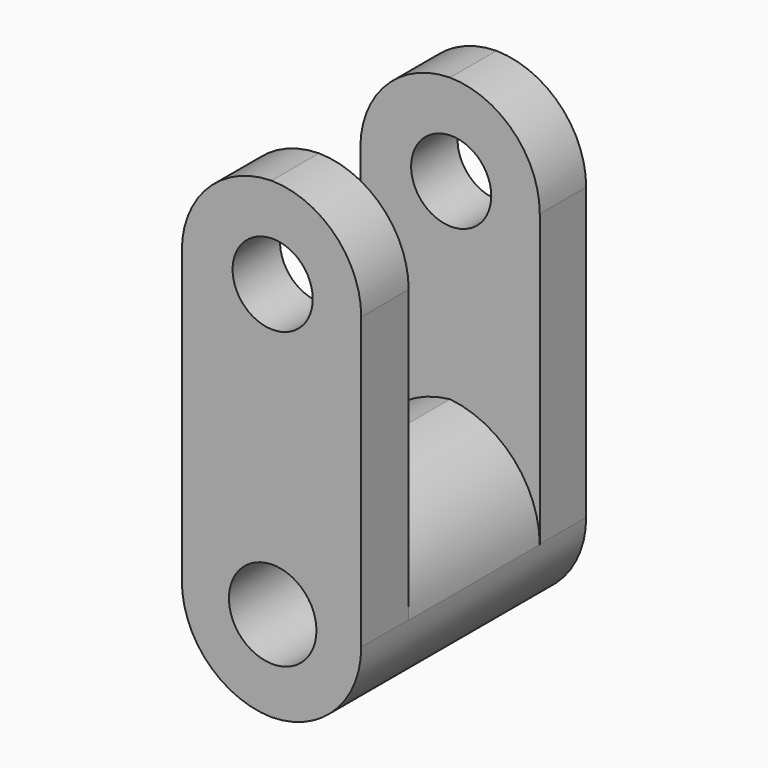
from build123d import *

# Parameters (mm, degrees)
F0_W        = 58.9435696602
F0_H        = 155.2014648914
F4_DEPTH    = 46.1890073493
F5_W        = 53.8340881467
F5_H        = 92.8563177586
F1_DEPTH    = 58.9445696602
F2_T1_DEPTH = 168.3050352459
F2_T3_DEPTH = 168.726075006
F2_T5_DEPTH = 241.6216065486
F3_T1_DEPTH = 53.8340881467
F6_R        = 13.164421927
F6_R_2      = 14.3764863779
F7_DEPTH    = 92.3790146986


# Not quite as in the source:
# - a fillet or chamfer that OpenCascade refuses, or shapes differently, is made with other operations: its cross-section is extruded or revolved along the edge and cut away or added


with BuildPart() as f4:
    # F0 (on Front) → F4 (new body, symmetric)
    with BuildSketch(Plane.XZ):
        Rectangle(F0_W, F0_H)
    extrude(amount=F4_DEPTH, both=True)

    # F5 (on face) → F1 (cut, through all)
    with BuildSketch(Plane.YZ.offset(29.4717848301)):
        with Locations((0.2105198801, 31.1725735664)):
            Rectangle(F5_W, F5_H)
    extrude(amount=-F1_DEPTH, mode=Mode.SUBTRACT)

    # F2: fillet of radius 29.84871837 on 6 edges, made by hand

    # F2_s2 → F2_t1 (cut)
    with BuildSketch(Plane.XZ.offset(-120.8108032743)):
        with BuildLine():
            ThreePointArc((29.4717848301, 47.7520140757), (20.7292976292, 68.8582452449), (-0.3769335399, 77.6007324457))
            Line((-0.3769335399, 77.6007324457), (29.4717848301, 77.6007324457))
            Line((29.4717848301, 77.6007324457), (29.4717848301, 47.7520140757))
        make_face()
        with BuildLine():
            ThreePointArc((-29.4717848301, 47.7520140757), (-20.7292976292, 68.8582452449), (0.3769335399, 77.6007324457))
            Line((0.3769335399, 77.6007324457), (-29.4717848301, 77.6007324457))
            Line((-29.4717848301, 77.6007324457), (-29.4717848301, 47.7520140757))
        make_face()
    extrude(amount=F2_T1_DEPTH, mode=Mode.SUBTRACT)

    # F2_s4 → F2_t3 (cut)
    with BuildSketch(Plane.XZ.offset(-47.9152717317)):
        with BuildLine():
            ThreePointArc((29.4717848301, 47.7520140757), (20.7292976292, 68.8582452449), (-0.3769335399, 77.6007324457))
            Line((-0.3769335399, 77.6007324457), (29.4717848301, 77.6007324457))
            Line((29.4717848301, 77.6007324457), (29.4717848301, 47.7520140757))
        make_face()
        with BuildLine():
            ThreePointArc((-29.4717848301, 47.7520140757), (-20.7292976292, 68.8582452449), (0.3769335399, 77.6007324457))
            Line((0.3769335399, 77.6007324457), (-29.4717848301, 77.6007324457))
            Line((-29.4717848301, 77.6007324457), (-29.4717848301, 47.7520140757))
        make_face()
    extrude(amount=F2_T3_DEPTH, mode=Mode.SUBTRACT)

    # F2_s6 → F2_t5 (cut)
    with BuildSketch(Plane.XZ.offset(-120.8108032743)):
        with BuildLine():
            ThreePointArc((-0.3769335399, -77.6007324457), (20.7292976292, -68.8582452449), (29.4717848301, -47.7520140757))
            Line((29.4717848301, -47.7520140757), (29.4717848301, -77.6007324457))
            Line((29.4717848301, -77.6007324457), (-0.3769335399, -77.6007324457))
        make_face()
        with BuildLine():
            ThreePointArc((0.3769335399, -77.6007324457), (-20.7292976292, -68.8582452449), (-29.4717848301, -47.7520140757))
            Line((-29.4717848301, -47.7520140757), (-29.4717848301, -77.6007324457))
            Line((-29.4717848301, -77.6007324457), (0.3769335399, -77.6007324457))
        make_face()
    extrude(amount=F2_T5_DEPTH, mode=Mode.SUBTRACT)

    # F3: fillet of radius 32.8509948239 on 2 edges, made by hand

    # F3_s2 → F3_t1 (cut)
    with BuildSketch(Plane.XZ.offset(-27.1275639534)):
        with BuildLine():
            ThreePointArc((29.4717848301, -48.1065801367), (19.8499512149, -24.877418928), (-3.3792099938, -15.2555853128))
            Line((-3.3792099938, -15.2555853128), (29.4717848301, -15.2555853128))
            Line((29.4717848301, -15.2555853128), (29.4717848301, -48.1065801367))
        make_face()
        with BuildLine():
            ThreePointArc((-29.4717848301, -48.1065801367), (-19.8499512149, -24.877418928), (3.3792099938, -15.2555853128))
            Line((3.3792099938, -15.2555853128), (-29.4717848301, -15.2555853128))
            Line((-29.4717848301, -15.2555853128), (-29.4717848301, -48.1065801367))
        make_face()
    extrude(amount=F3_T1_DEPTH, mode=Mode.SUBTRACT)

    # F6 (on face) → F7 (cut, through all)
    with BuildSketch(Plane.XZ.offset(46.1890073493)):
        with Locations((0.3769335399, 47.7520140757)):
            Circle(F6_R)
        with Locations((0.3769335399, -47.7520140757)):
            Circle(F6_R_2)
    extrude(amount=-F7_DEPTH, mode=Mode.SUBTRACT)


solid = f4.part
